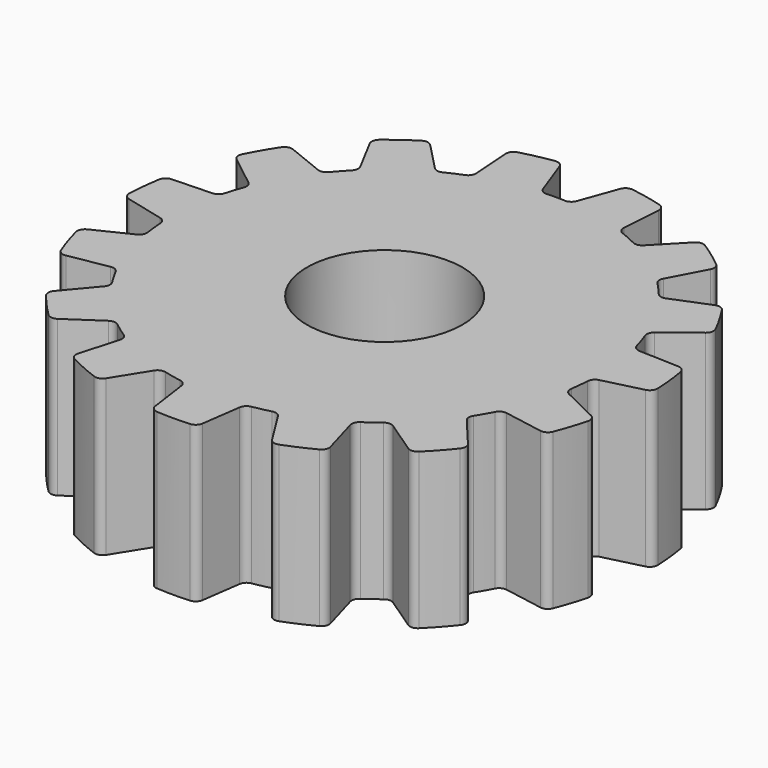
from build123d import *

# Parameters (mm, degrees)
F0_R            = 8.5
F0_R_2          = 2.5
F1_DEPTH        = 5
F3_DEPTH        = 25
F3_COPIES_COUNT = 15
F4_R            = 0.25


# Not quite as in the source:
# - a feature of the source that left no trace in its solid (it failed there, or was rolled back) is left out
# - a pattern or mirror of a feature is missing from the dataset's text; its kind, count and spacing are read off the source's solid


with BuildPart() as f1:
    # F0 (on Top) → F1 (new body)
    with BuildSketch(Plane.XY):
        Circle(F0_R)
        Circle(F0_R_2, mode=Mode.SUBTRACT)
    extrude(amount=F1_DEPTH)

    # F2 (on face) → F3 (cut)
    with BuildSketch(Plane.XY.offset(5)):
        with BuildLine():
            ThreePointArc((-0.4741372428, 6.8656537447), (0, 6.8820060641), (0.4741372428, 6.8656537447))
            Line((0.4741372428, 6.8656537447), (1.0454988446, 8.4354568439))
            ThreePointArc((1.0454988446, 8.4354568439), (0, 8.5), (-1.0454988446, 8.4354568439))
            Line((-1.0454988446, 8.4354568439), (-0.4741372428, 6.8656537447))
        make_face()
    f3 = extrude(amount=-F3_DEPTH, mode=Mode.SUBTRACT)

    # F3_copies: F3 ×15 about axis
    f3_copies_axis = Axis((0, 0, 0), (0, 0, 1))
    for i in range(1, F3_COPIES_COUNT):
        add(f3.rotate(f3_copies_axis, i * 360 / F3_COPIES_COUNT), mode=Mode.SUBTRACT)

    # F4
    f4_edges = [f1.edges().sort_by_distance(p)[0] for p in [
        (-0.474137, 6.865654, 2.5),
        (-1.045499, 8.435457, 2.5),
        (0.474137, 6.865654, 2.5),
        (1.045499, 8.435457, 2.5),
        (-2.475899, 8.131416, 2.5),
        (-2.359367, 6.464936, 2.5),
        (2.475899, 8.131416, 2.5),
        (2.359367, 6.464936, 2.5),
        (3.225659, 6.079238, 2.5),
        (4.38612, 7.280931, 2.5),
        (5.569191, 6.421379, 2.5),
        (4.784915, 4.946372, 2.5),
        (5.419435, 4.241666, 2.5),
        (6.968341, 4.867465, 2.5),
        (7.699519, 3.601028, 2.5),
        (6.383108, 2.572535, 2.5),
        (6.676141, 1.670672, 2.5),
        (8.345673, 1.612371, 2.5),
        (8.498531, 0.158026, 2.5),
        (6.877604, -0.246116, 2.5),
        (6.778482, -1.189196, 2.5),
        (8.279962, -1.921517, 2.5),
        (7.828069, -3.3123, 2.5),
        (6.182899, -3.022212, 2.5),
        (5.708762, -3.843442, 2.5),
        (6.78257, -5.123157, 2.5),
        (5.804063, -6.209899, 2.5),
        (4.419115, -5.27574, 2.5),
        (3.651945, -5.833121, 2.5),
        (4.112411, -7.438957, 2.5),
        (2.776482, -8.03375, 2.5),
        (1.891226, -6.617044, 2.5),
        (0.963673, -6.814201, 2.5),
        (0.731178, -8.468493, 2.5),
        (-0.731178, -8.468493, 2.5),
        (-0.963673, -6.814201, 2.5),
        (-1.891226, -6.617044, 2.5),
        (-2.776482, -8.03375, 2.5),
        (-4.112411, -7.438957, 2.5),
        (-3.651945, -5.833121, 2.5),
        (-4.419115, -5.27574, 2.5),
        (-5.804063, -6.209899, 2.5),
        (-6.78257, -5.123157, 2.5),
        (-5.708762, -3.843442, 2.5),
        (-6.182899, -3.022212, 2.5),
        (-7.828069, -3.3123, 2.5),
        (-8.279962, -1.921517, 2.5),
        (-6.778482, -1.189196, 2.5),
        (-6.877604, -0.246116, 2.5),
        (-8.498531, 0.158026, 2.5),
        (-8.345673, 1.612371, 2.5),
        (-6.676141, 1.670672, 2.5),
        (-6.383108, 2.572535, 2.5),
        (-7.699519, 3.601028, 2.5),
        (-6.968341, 4.867465, 2.5),
        (-5.419435, 4.241666, 2.5),
        (-4.784915, 4.946372, 2.5),
        (-5.569191, 6.421379, 2.5),
        (-4.38612, 7.280931, 2.5),
        (-3.225659, 6.079238, 2.5),
    ]]
    fillet(f4_edges, radius=F4_R)


solid = f1.part
